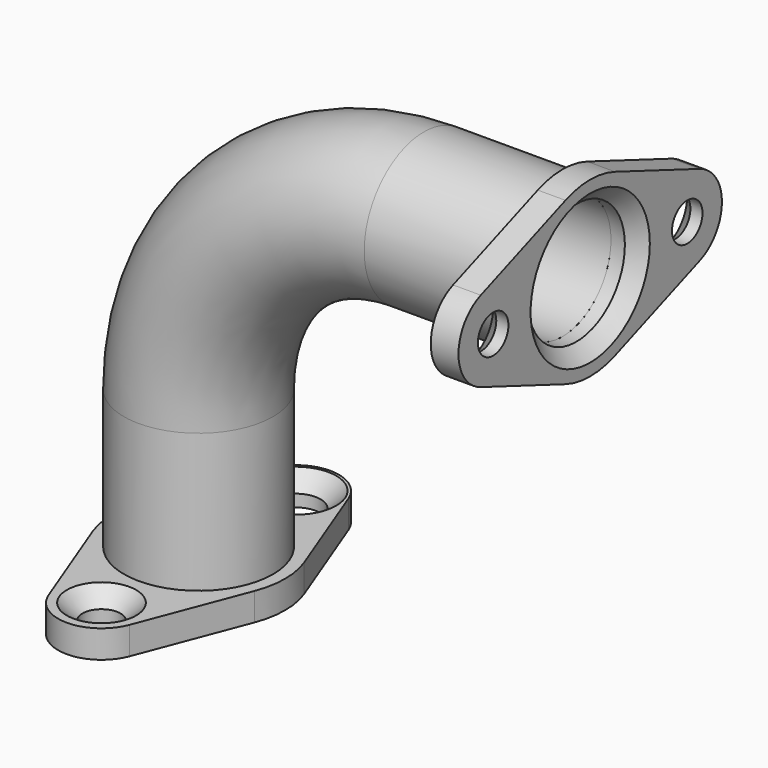
from build123d import *

# Parameters (mm, degrees)
F1_R      = 21.5
F1_R_2    = 17.5
F3_R      = 7.2092670895
F3_R_2    = 21.5
F3_R_3    = 5.5
F3_R_4    = 17.5
F4_DEPTH  = 8
F5_R      = 5.5
F5_R_2    = 21.5
F5_R_3    = 17.5
F6_DEPTH  = 8
F7_SIZE   = 4.5
F7_2_SIZE = 4.5
F8_SIZE   = 4
F8_2_SIZE = 4


with BuildPart() as f2:
    # F2: sweep along a path in F0
    with BuildLine(Plane.XZ) as f2_path:
        Line((-65, -40), (-65, 0))
        ThreePointArc((-65, 0), (-45.9619407771, 45.9619407771), (0, 65))
        Line((0, 65), (40, 65))
    # F1 (on Top) → F2 (sweep)
    with BuildSketch(Plane.XY):
        with Locations((-65, 0)):
            Circle(F1_R)
        with Locations((-65, 0)):
            Circle(F1_R_2, mode=Mode.SUBTRACT)
    sweep(path=f2_path.line)


with BuildPart() as f4:
    # F3 (on face) → F4 (new body)
    with BuildSketch(Plane(origin=(0, 0, -40), x_dir=(1, 0, 0), z_dir=(0, 0, -1))):
        with BuildLine():
            Line((-76.6756221702, 39.4642857143), (-88.3512443404, 8.9285714286))
            ThreePointArc((-88.3512443404, 8.9285714286), (-90, 0), (-88.3512443404, -8.9285714286))
            Line((-88.3512443404, -8.9285714286), (-76.6756221702, -39.4642857143))
            ThreePointArc((-76.6756221702, -39.4642857143), (-65, -47.5), (-53.3243778298, -39.4642857143))
            Line((-53.3243778298, -39.4642857143), (-41.6487556596, -8.9285714286))
            ThreePointArc((-41.6487556596, -8.9285714286), (-40, 0), (-41.6487556596, 8.9285714286))
            Line((-41.6487556596, 8.9285714286), (-53.3243778298, 39.4642857143))
            ThreePointArc((-53.3243778298, 39.4642857143), (-65, 47.5), (-76.6756221702, 39.4642857143))
        make_face()
        with Locations((-65, -35)):
            Circle(F3_R, mode=Mode.SUBTRACT)
        with Locations((-65, 0)):
            Circle(F3_R_2, mode=Mode.SUBTRACT)
        with Locations((-65, 35)):
            Circle(F3_R_3, mode=Mode.SUBTRACT)
        with Locations((-65, 0)):
            Circle(F3_R_2)
        with Locations((-65, 0)):
            Circle(F3_R_4, mode=Mode.SUBTRACT)
    extrude(amount=F4_DEPTH)

    # F7
    f7_edges = [f4.edges().sort_by_distance(p)[0] for p in [
        (-72.209267, 35, -40),
        (-70.5, -35, -40),
    ]]
    chamfer(f7_edges, length=F7_SIZE)

    # F8
    f8_edges = [f4.edges().sort_by_distance(p)[0] for p in [
        (-82.5, 0, -48),
    ]]
    chamfer(f8_edges, length=F8_SIZE)


with BuildPart() as f6:
    # F5 (on face) → F6 (new body)
    with BuildSketch(Plane.YZ.offset(40)):
        with BuildLine():
            Line((39.4642857143, 76.6756221702), (8.9285714286, 88.3512443404))
            ThreePointArc((8.9285714286, 88.3512443404), (0, 90), (-8.9285714286, 88.3512443404))
            Line((-8.9285714286, 88.3512443404), (-39.4642857143, 76.6756221702))
            ThreePointArc((-39.4642857143, 76.6756221702), (-47.5, 65), (-39.4642857143, 53.3243778298))
            Line((-39.4642857143, 53.3243778298), (-8.9285714286, 41.6487556596))
            ThreePointArc((-8.9285714286, 41.6487556596), (0, 40), (8.9285714286, 41.6487556596))
            Line((8.9285714286, 41.6487556596), (39.4642857143, 53.3243778298))
            ThreePointArc((39.4642857143, 53.3243778298), (47.5, 65), (39.4642857143, 76.6756221702))
        make_face()
        with Locations((-35, 65)):
            Circle(F5_R, mode=Mode.SUBTRACT)
        with Locations((0, 65)):
            Circle(F5_R_2, mode=Mode.SUBTRACT)
        with Locations((35, 65)):
            Circle(F5_R, mode=Mode.SUBTRACT)
        with Locations((0, 65)):
            Circle(F5_R_2)
        with Locations((0, 65)):
            Circle(F5_R_3, mode=Mode.SUBTRACT)
    extrude(amount=F6_DEPTH)

    # F7#2
    f7_2_edges = [f6.edges().sort_by_distance(p)[0] for p in [
        (40, 29.5, 65),
        (40, -40.5, 65),
    ]]
    chamfer(f7_2_edges, length=F7_2_SIZE)

    # F8#2
    f8_2_edges = [f6.edges().sort_by_distance(p)[0] for p in [
        (48, -17.5, 65),
    ]]
    chamfer(f8_2_edges, length=F8_2_SIZE)


solid = Compound([f2.part, f4.part, f6.part])
